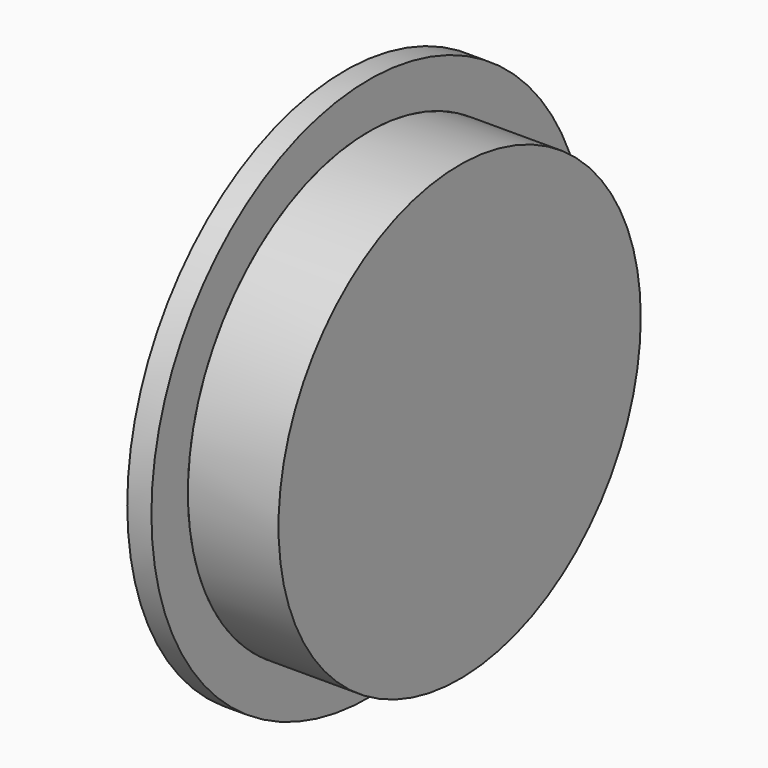
from build123d import *

# Parameters (mm, degrees)
F0_R     = 15.8665178104
F1_DEPTH = 6.35
F2_R     = 19.064952095
F2_R_2   = 15.8665178104
F3_DEPTH = 1.6933333333


# Not quite as in the source:
# - a length typed as a fraction of an inch, garbled in the dataset ("3 / 203.2 mm" for 3/8 in), is restored


with BuildPart() as f1:
    # F0 (on Right) → F1 (new body)
    with BuildSketch(Plane.YZ):
        Circle(F0_R)
    extrude(amount=F1_DEPTH)


with BuildPart() as f3:
    # F2 (on face) → F3 (new body)
    with BuildSketch(Plane(origin=(0, 0, 0), x_dir=(0, -1, 0), z_dir=(-1, 0, 0))):
        Circle(F2_R)
        Circle(F2_R_2, mode=Mode.SUBTRACT)
    extrude(amount=F3_DEPTH)


solid = Compound([f1.part, f3.part])
